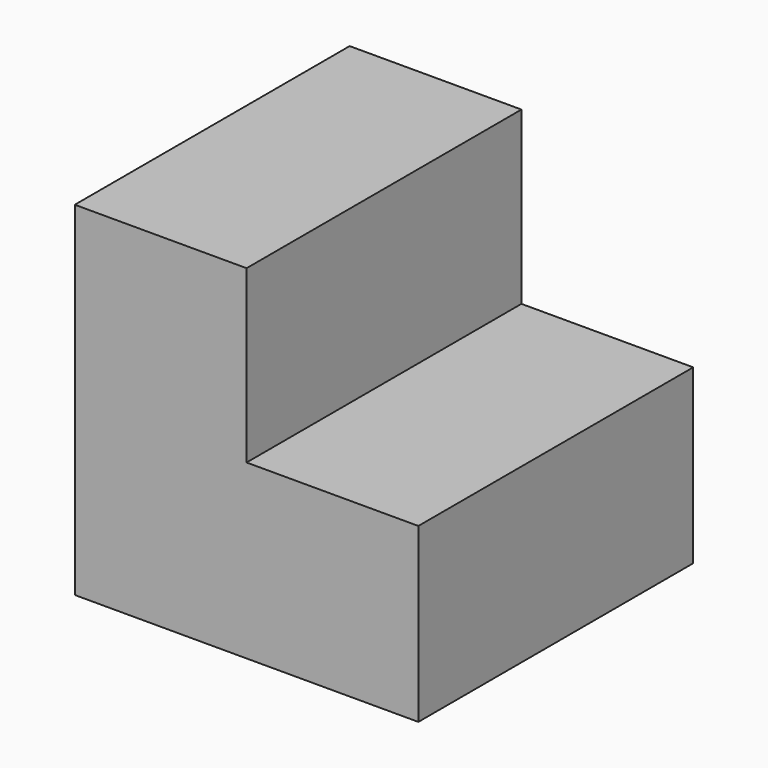
from build123d import *

# Parameters (mm, degrees)
F1_DEPTH = 100


# Not quite as in the source:
# - a feature names something its author has since deleted; it is built from what else it names


with BuildPart() as f1:
    # F0 (on Front) → F1 (new body)
    with BuildSketch(Plane.XZ):
        Polygon((50, 115.3164558689), (0, 115.3164558689), (0, 15.3164558689), (100, 15.3164558689), (100, 65.5276626348), (50, 65.5276626348), align=None)
    extrude(amount=-F1_DEPTH)


solid = f1.part
